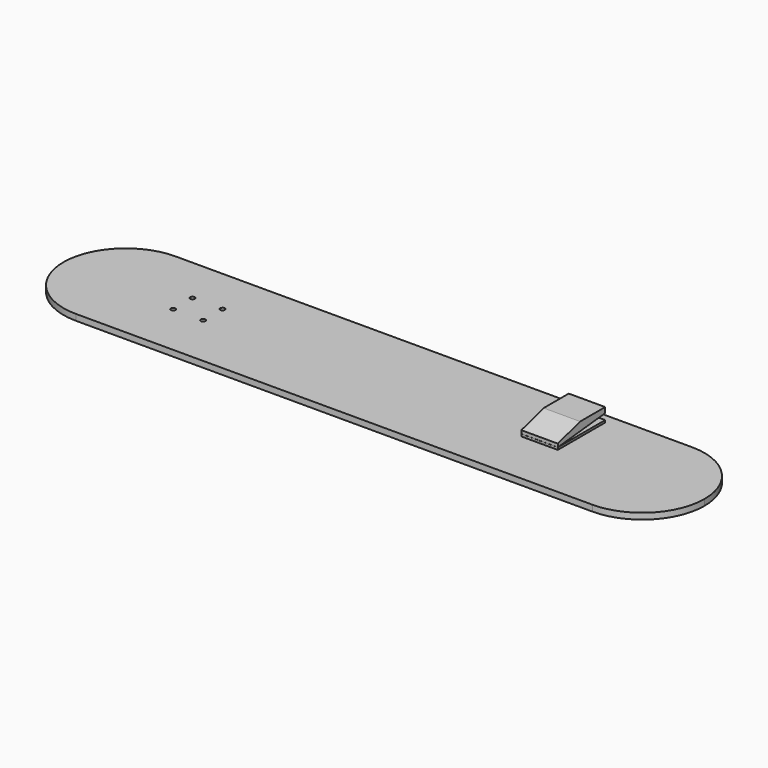
from build123d import *

# Parameters (mm, degrees)
F0_W     = 863.6
F0_H     = 208.28
F1_DEPTH = 10.16
F3_DEPTH = 33.02
F5_DEPTH = 734.06
F6_DEPTH = 548.64


# Not quite as in the source:
# - a feature names something its author has since deleted; it is built from what else it names


with BuildPart() as f1:
    # F0 (on Top) → F1 (new body)
    with BuildSketch(Plane.XY):
        Rectangle(F0_W, F0_H)
        with BuildLine():
            ThreePointArc((-337.1454958344, -14.4779989496), (-343.6495726707, -17.1720757859), (-340.9554958344, -10.6679989496))
            ThreePointArc((-340.9554958344, -10.6679989496), (-338.261418998, -11.7839221133), (-337.1454958344, -14.4779989496))
        make_face(mode=Mode.SUBTRACT)
        with BuildLine():
            ThreePointArc((-287.1074958344, -14.4779989496), (-293.6115726707, -17.1720757859), (-290.9174958344, -10.6679989496))
            ThreePointArc((-290.9174958344, -10.6679989496), (-288.223418998, -11.7839221133), (-287.1074958344, -14.4779989496))
        make_face(mode=Mode.SUBTRACT)
        with BuildLine():
            ThreePointArc((-340.9554958344, 22.3520010504), (-343.6495726707, 28.8560778867), (-337.1454958344, 26.1620010504))
            ThreePointArc((-337.1454958344, 26.1620010504), (-338.261418998, 23.4679242141), (-340.9554958344, 22.3520010504))
        make_face(mode=Mode.SUBTRACT)
        with BuildLine():
            ThreePointArc((-290.9174958344, 22.3520010504), (-293.6115726707, 23.4679242141), (-294.7274958344, 26.1620010504))
            ThreePointArc((-294.7274958344, 26.1620010504), (-290.9174958344, 29.9720010504), (-287.1074958344, 26.1620010504))
            ThreePointArc((-287.1074958344, 26.1620010504), (-288.223418998, 23.4679242141), (-290.9174958344, 22.3520010504))
        make_face(mode=Mode.SUBTRACT)
        with BuildLine():
            ThreePointArc((-535.94, 0), (-505.4381001928, -73.6381001928), (-431.8, -104.14))
            Line((-431.8, -104.14), (-431.8, 104.14))
            ThreePointArc((-431.8, 104.14), (-505.4381001928, 73.6381001928), (-535.94, 0))
        make_face()
        with BuildLine():
            Line((431.8, 104.14), (431.8, -104.14))
            ThreePointArc((431.8, -104.14), (505.4381001928, -73.6381001928), (535.94, 0))
            ThreePointArc((535.94, 0), (505.4381001928, 73.6381001928), (431.8, 104.14))
        make_face()
    extrude(amount=F1_DEPTH)

    # F2 (on Top) → F3 (join)
    with BuildSketch(Plane.XY):
        Polygon((238.76, -11.43), (299.72, -11.43), (299.72, 87.63), (238.76, 87.63), (238.76, 0), align=None)
    extrude(amount=F3_DEPTH)

    # F4 (on Right) → F5 (cut)
    with BuildSketch(Plane.YZ):
        Polygon((-16.7762897909, 37.7759821713), (-15.3684904799, 18.3014087379), (51.5020377934, 37.7759821713), align=None)
        Polygon((93.5014262795, 24.6365107596), (-12.7875227481, 13.8433724642), (93.5014262795, 13.8433724642), align=None)
    extrude(amount=F5_DEPTH, mode=Mode.SUBTRACT)

    # F0 (on Top) → F6 (cut)
    with BuildSketch(Plane.XY):
        Rectangle(F0_W, F0_H)
        with BuildLine():
            ThreePointArc((-337.1454958344, -14.4779989496), (-343.6495726707, -17.1720757859), (-340.9554958344, -10.6679989496))
            ThreePointArc((-340.9554958344, -10.6679989496), (-338.261418998, -11.7839221133), (-337.1454958344, -14.4779989496))
        make_face(mode=Mode.SUBTRACT)
        with BuildLine():
            ThreePointArc((-287.1074958344, -14.4779989496), (-293.6115726707, -17.1720757859), (-290.9174958344, -10.6679989496))
            ThreePointArc((-290.9174958344, -10.6679989496), (-288.223418998, -11.7839221133), (-287.1074958344, -14.4779989496))
        make_face(mode=Mode.SUBTRACT)
        with BuildLine():
            ThreePointArc((-340.9554958344, 22.3520010504), (-343.6495726707, 28.8560778867), (-337.1454958344, 26.1620010504))
            ThreePointArc((-337.1454958344, 26.1620010504), (-338.261418998, 23.4679242141), (-340.9554958344, 22.3520010504))
        make_face(mode=Mode.SUBTRACT)
        with BuildLine():
            ThreePointArc((-290.9174958344, 22.3520010504), (-293.6115726707, 23.4679242141), (-294.7274958344, 26.1620010504))
            ThreePointArc((-294.7274958344, 26.1620010504), (-290.9174958344, 29.9720010504), (-287.1074958344, 26.1620010504))
            ThreePointArc((-287.1074958344, 26.1620010504), (-288.223418998, 23.4679242141), (-290.9174958344, 22.3520010504))
        make_face(mode=Mode.SUBTRACT)
        with BuildLine():
            ThreePointArc((-535.94, 0), (-505.4381001928, -73.6381001928), (-431.8, -104.14))
            Line((-431.8, -104.14), (-431.8, 104.14))
            ThreePointArc((-431.8, 104.14), (-505.4381001928, 73.6381001928), (-535.94, 0))
        make_face()
        with BuildLine():
            Line((431.8, 104.14), (431.8, -104.14))
            ThreePointArc((431.8, -104.14), (505.4381001928, -73.6381001928), (535.94, 0))
            ThreePointArc((535.94, 0), (505.4381001928, 73.6381001928), (431.8, 104.14))
        make_face()
    extrude(amount=-F6_DEPTH, mode=Mode.SUBTRACT)


solid = f1.part
